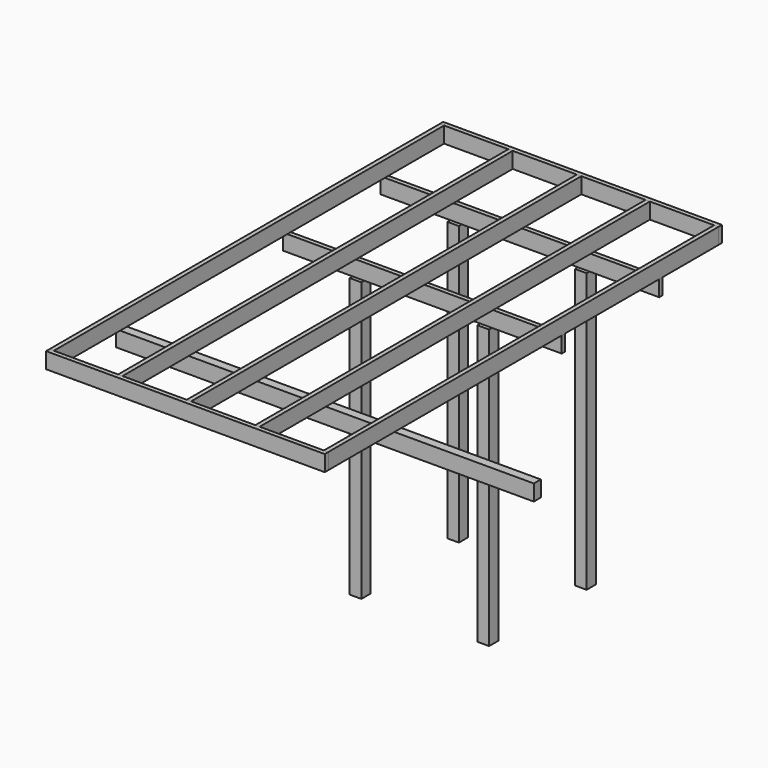
from build123d import *

# Parameters (mm, degrees)
F0_W     = 101.6
F0_H     = 31.75
F1_DEPTH = 2438.4
F0_H_2   = 38.1
F0_W_2   = 1016
F0_W_3   = 609.6
F2_DEPTH = 139.7
F0_W_4   = 3657.6
F0_H_3   = 76.2
F4_DEPTH = 139.7
F3_W     = 38.1
F3_H     = 3619.5
F3_H_2   = 38.1
F3_H_3   = 609.6
F5_DEPTH = 139.7


with BuildPart() as f1:
    # F0 (on Top) → F1 (new body)
    with BuildSketch(Plane.XY):
        with Locations((-687.2804223888, 137.6850830514)):
            Rectangle(F0_W, F0_H)
        Polygon((-636.4804223888, 121.8100830514), (-738.0804223888, 121.8100830514), (-738.0804223888, 102.7600830514), (-738.0804223888, 83.7100830514), (-636.4804223888, 83.7100830514), align=None)
        with Locations((-687.2804223888, 67.8350830514)):
            Rectangle(F0_W, F0_H)
    extrude(amount=-F1_DEPTH)


with BuildPart() as f1b:
    # F0 (on Top) → F1, piece 2 (new body)
    with BuildSketch(Plane.XY):
        with Locations((430.3195776112, 102.7600830514)):
            Rectangle(F0_W, F0_H_2)
        with Locations((430.3195776112, 137.6850830514)):
            Rectangle(F0_W, F0_H)
        with Locations((430.3195776112, 67.8350830514)):
            Rectangle(F0_W, F0_H)
    extrude(amount=-F1_DEPTH)


with BuildPart() as f1c:
    # F0 (on Top) → F1, piece 3 (new body)
    with BuildSketch(Plane.XY):
        with Locations((430.3195776112, -929.1149169486)):
            Rectangle(F0_W, F0_H)
        with Locations((430.3195776112, -964.0399169486)):
            Rectangle(F0_W, F0_H_2)
        with Locations((430.3195776112, -998.9649169486)):
            Rectangle(F0_W, F0_H)
    extrude(amount=-F1_DEPTH)


with BuildPart() as f1d:
    # F0 (on Top) → F1, piece 4 (new body)
    with BuildSketch(Plane.XY):
        Polygon((-636.4804223888, -983.0899169486), (-636.4804223888, -944.9899169486), (-738.0804223888, -944.9899169486), (-738.0804223888, -964.0399169486), (-738.0804223888, -983.0899169486), align=None)
        with Locations((-687.2804223888, -929.1149169486)):
            Rectangle(F0_W, F0_H)
        with Locations((-687.2804223888, -998.9649169486)):
            Rectangle(F0_W, F0_H)
    extrude(amount=-F1_DEPTH)


with BuildPart() as f2:
    # F0 (on Top) → F2 (new body)
    with BuildSketch(Plane.XY):
        Polygon((-636.4804223888, 121.8100830514), (-738.0804223888, 121.8100830514), (-738.0804223888, 102.7600830514), (-738.0804223888, 83.7100830514), (-636.4804223888, 83.7100830514), align=None)
        Polygon((-738.0804223888, 102.7600830514), (-738.0804223888, 121.8100830514), (-1347.6804223888, 121.8100830514), (-1347.6804223888, 83.7100830514), (-738.0804223888, 83.7100830514), align=None)
        with Locations((-128.4804223888, 102.7600830514)):
            Rectangle(F0_W_2, F0_H_2)
        with Locations((430.3195776112, 102.7600830514)):
            Rectangle(F0_W, F0_H_2)
        with Locations((785.9195776112, 102.7600830514)):
            Rectangle(F0_W_3, F0_H_2)
    extrude(amount=F2_DEPTH)


with BuildPart() as f2b:
    # F0 (on Top) → F2, piece 2 (new body)
    with BuildSketch(Plane.XY):
        with Locations((785.9195776112, -964.0399169486)):
            Rectangle(F0_W_3, F0_H_2)
        with Locations((430.3195776112, -964.0399169486)):
            Rectangle(F0_W, F0_H_2)
        with Locations((-128.4804223888, -964.0399169486)):
            Rectangle(F0_W_2, F0_H_2)
        Polygon((-636.4804223888, -983.0899169486), (-636.4804223888, -944.9899169486), (-738.0804223888, -944.9899169486), (-738.0804223888, -964.0399169486), (-738.0804223888, -983.0899169486), align=None)
        Polygon((-738.0804223888, -964.0399169486), (-738.0804223888, -944.9899169486), (-1347.6804223888, -944.9899169486), (-1347.6804223888, -983.0899169486), (-738.0804223888, -983.0899169486), align=None)
    extrude(amount=F2_DEPTH)


with BuildPart() as f2c:
    # F0 (on Top) → F2, piece 3 (new body)
    with BuildSketch(Plane.XY):
        with Locations((481.1195776112, -2773.7899169486)):
            Rectangle(F0_W_4, F0_H_3)
    extrude(amount=F2_DEPTH)


with BuildPart() as f4:
    # F3 (on face) → F4 (new body)
    with BuildSketch(Plane.XY.offset(139.7)):
        Polygon((-1347.6804223888, 769.5100830514), (-1347.6804223888, 731.4100830514), (-1309.5804223888, 731.4100830514), (-747.6054223888, 731.4100830514), (-709.5054223888, 731.4100830514), (-147.5304223888, 731.4100830514), (-109.4304223888, 731.4100830514), (452.5445776112, 731.4100830514), (490.6445776112, 731.4100830514), (1052.6195776112, 731.4100830514), (1090.7195776112, 731.4100830514), (1090.7195776112, 769.5100830514), align=None)
    extrude(amount=F4_DEPTH)


with BuildPart() as f4b:
    # F3 (on face) → F4, piece 2 (new body)
    with BuildSketch(Plane.XY.offset(139.7)):
        Polygon((-1309.5804223888, -3535.7899169486), (-1347.6804223888, -3535.7899169486), (-1347.6804223888, -3573.8899169486), (1090.7195776112, -3573.8899169486), (1090.7195776112, -3535.7899169486), (1052.6195776112, -3535.7899169486), (490.6445776112, -3535.7899169486), (452.5445776112, -3535.7899169486), (-109.4304223888, -3535.7899169486), (-147.5304223888, -3535.7899169486), (-709.5054223888, -3535.7899169486), (-747.6054223888, -3535.7899169486), align=None)
    extrude(amount=F4_DEPTH)


with BuildPart() as f5:
    # F3 (on face) → F5 (new body)
    with BuildSketch(Plane.XY.offset(139.7)):
        with Locations((-1328.6304223888, -1726.0399169486)):
            Rectangle(F3_W, F3_H)
        with Locations((-1328.6304223888, 102.7600830514)):
            Rectangle(F3_W, F3_H_2)
        with Locations((-1328.6304223888, 426.6100830514)):
            Rectangle(F3_W, F3_H_3)
    extrude(amount=F5_DEPTH)


with BuildPart() as f5b:
    # F3 (on face) → F5, piece 2 (new body)
    with BuildSketch(Plane.XY.offset(139.7)):
        with Locations((-728.5554223888, -1726.0399169486)):
            Rectangle(F3_W, F3_H)
        with Locations((-728.5554223888, 426.6100830514)):
            Rectangle(F3_W, F3_H_3)
        with Locations((-728.5554223888, 102.7600830514)):
            Rectangle(F3_W, F3_H_2)
    extrude(amount=F5_DEPTH)


with BuildPart() as f5c:
    # F3 (on face) → F5, piece 3 (new body)
    with BuildSketch(Plane.XY.offset(139.7)):
        with Locations((-128.4804223888, -1726.0399169486)):
            Rectangle(F3_W, F3_H)
        with Locations((-128.4804223888, 102.7600830514)):
            Rectangle(F3_W, F3_H_2)
        with Locations((-128.4804223888, 426.6100830514)):
            Rectangle(F3_W, F3_H_3)
    extrude(amount=F5_DEPTH)


with BuildPart() as f5d:
    # F3 (on face) → F5, piece 4 (new body)
    with BuildSketch(Plane.XY.offset(139.7)):
        with Locations((471.5945776112, -1726.0399169486)):
            Rectangle(F3_W, F3_H)
        with Locations((471.5945776112, 426.6100830514)):
            Rectangle(F3_W, F3_H_3)
        with Locations((471.5945776112, 102.7600830514)):
            Rectangle(F3_W, F3_H_2)
    extrude(amount=F5_DEPTH)


with BuildPart() as f5e:
    # F3 (on face) → F5, piece 5 (new body)
    with BuildSketch(Plane.XY.offset(139.7)):
        with Locations((1071.6695776112, -1726.0399169486)):
            Rectangle(F3_W, F3_H)
        with Locations((1071.6695776112, 426.6100830514)):
            Rectangle(F3_W, F3_H_3)
        with Locations((1071.6695776112, 102.7600830514)):
            Rectangle(F3_W, F3_H_2)
    extrude(amount=F5_DEPTH)


solid = Compound([f1.part, f1b.part, f1c.part, f1d.part, f2.part, f2b.part, f2c.part, f4.part, f4b.part, f5.part, f5b.part, f5c.part, f5d.part, f5e.part])
